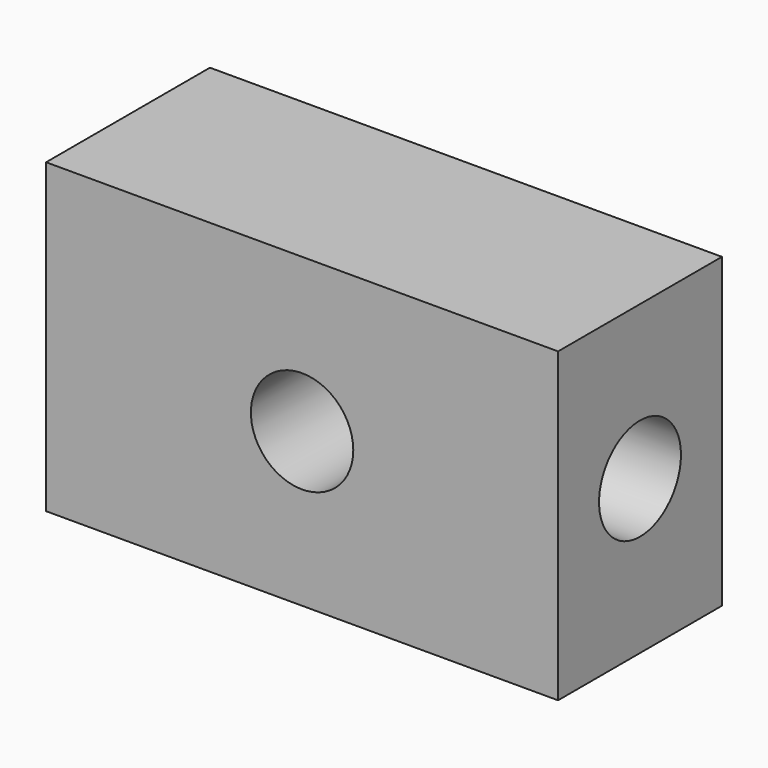
from build123d import *

# Parameters (mm, degrees)
F0_W          = 127
F0_H          = 76.2
F1_DEPTH      = 25.4
F1_DEPTH_BACK = 25.4
F2_R          = 12.7
F3_DEPTH      = 44.45
F4_R          = 12.7
F5_DEPTH      = 44.45


# Not quite as in the source:
# - a feature names something its author has since deleted; it is built from what else it names


with BuildPart() as f1:
    # F0 (on Front) → F1 (new body, two sides)
    with BuildSketch(Plane.XZ) as f1_sk:
        with Locations((1.2215264142, -26.8060624134)):
            Rectangle(F0_W, F0_H)
    extrude(amount=F1_DEPTH)
    extrude(f1_sk.sketch, amount=-F1_DEPTH_BACK)

    # F2 (on face) → F3 (cut)
    with BuildSketch(Plane.XZ.offset(25.4)):
        with Locations((1.2215264142, -26.8060624134)):
            Circle(F2_R)
    extrude(amount=-F3_DEPTH, mode=Mode.SUBTRACT)

    # F4 (on face) → F5 (cut)
    with BuildSketch(Plane.YZ.offset(64.7215264142)):
        with Locations((0, -26.8060624134)):
            Circle(F4_R)
    extrude(amount=-F5_DEPTH, mode=Mode.SUBTRACT)


solid = f1.part
